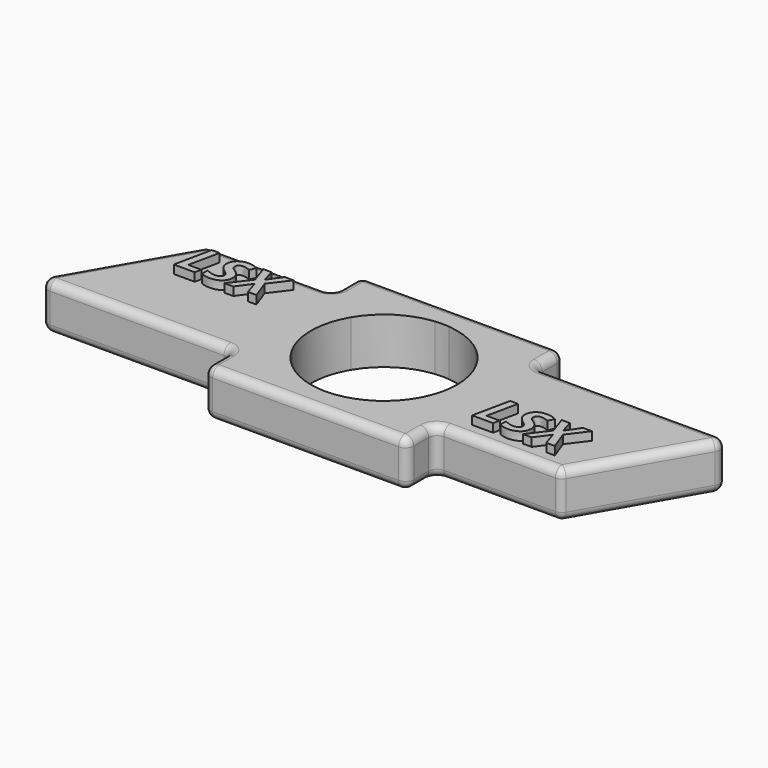
from build123d import *

# Parameters (mm, degrees)
F1_DEPTH     = 6.985
F2_TEXT_SIZE = 7.9375
F3_DEPTH     = 1.27
F4_R         = 1.27
F5_R         = 1.27
F6_R         = 1.27


# Not quite as in the source:
# - Text() gives the source's letters only with a copy of the font that has no kerning and outlines rounded to 1/6400 em; it was checked with that copy


with BuildPart() as f1:
    # F0 (on Top) → F1 (new body)
    with BuildSketch(Plane.XY):
        Polygon((-34.1459329325, 9.4483174), (-44.9994729931, -9.4487963283), (-15.3035, -9.4487963283), (-15.3035, -14.7827963283), (15.3035, -14.7827963283), (15.3035, -9.4487963283), (34.1459329325, -9.4487963283), (44.9994729931, 9.4483174), (15.3035, 9.4483174), (15.3035, 14.7823174), (-15.3035, 14.7823174), (-15.3035, 9.4483174), align=None)
        with BuildLine():
            Line((-11.4935, -5.6387963283), (-38.4175, -5.6387963283))
            Line((-38.4175, -5.6387963283), (-31.9405, 5.6383174))
            Line((-31.9405, 5.6383174), (-11.4935, 5.6383174))
            Line((-11.4935, 5.6383174), (-11.4935, 10.9723174))
            Line((-11.4935, 10.9723174), (-1.0620771317, 10.9723174))
            ThreePointArc((-1.0620771317, 10.9723174), (0, 11.0236), (1.0620771317, 10.9723174))
            Line((1.0620771317, 10.9723174), (11.4935, 10.9723174))
            Line((11.4935, 10.9723174), (11.4935, 5.6383174))
            Line((11.4935, 5.6383174), (38.4175, 5.6383174))
            Line((38.4175, 5.6383174), (31.9405, -5.6387963283))
            Line((31.9405, -5.6387963283), (11.4935, -5.6387963283))
            Line((11.4935, -5.6387963283), (11.4935, -10.9727963283))
            Line((11.4935, -10.9727963283), (1.0571176371, -10.9727963283))
            ThreePointArc((1.0571176371, -10.9727963283), (0, -11.0236), (-1.0571176371, -10.9727963283))
            Line((-1.0571176371, -10.9727963283), (-11.4935, -10.9727963283))
            Line((-11.4935, -10.9727963283), (-11.4935, -5.6387963283))
        make_face(mode=Mode.SUBTRACT)
        with BuildLine():
            Line((-31.9405, 5.6383174), (-38.4175, -5.6387963283))
            Line((-38.4175, -5.6387963283), (-11.4935, -5.6387963283))
            Line((-11.4935, -5.6387963283), (-11.4935, -10.9727963283))
            Line((-11.4935, -10.9727963283), (-1.0571176371, -10.9727963283))
            ThreePointArc((-1.0571176371, -10.9727963283), (-9.8336529635, -4.9818697649), (-9.4725463238, 5.6383174))
            Line((-9.4725463238, 5.6383174), (-11.4935, 5.6383174))
            Line((-11.4935, 5.6383174), (-31.9405, 5.6383174))
        make_face()
        with BuildLine():
            Line((-11.4935, 10.9723174), (-11.4935, 5.6383174))
            Line((-11.4935, 5.6383174), (-9.4725463238, 5.6383174))
            ThreePointArc((-9.4725463238, 5.6383174), (-5.9040208195, 9.30925857), (-1.0620771317, 10.9723174))
            Line((-1.0620771317, 10.9723174), (-11.4935, 10.9723174))
        make_face()
        with BuildLine():
            ThreePointArc((11.0236, 0), (8.1600551145, -7.4116973419), (1.0571176371, -10.9727963283))
            Line((1.0571176371, -10.9727963283), (11.4935, -10.9727963283))
            Line((11.4935, -10.9727963283), (11.4935, -5.6387963283))
            Line((11.4935, -5.6387963283), (31.9405, -5.6387963283))
            Line((31.9405, -5.6387963283), (38.4175, 5.6383174))
            Line((38.4175, 5.6383174), (11.4935, 5.6383174))
            Line((11.4935, 5.6383174), (11.4935, 10.9723174))
            Line((11.4935, 10.9723174), (1.0620771317, 10.9723174))
            ThreePointArc((1.0620771317, 10.9723174), (8.1617299156, 7.4098530178), (11.0236, 0))
        make_face()
    extrude(amount=F1_DEPTH)

    # F2 (on face) → F3 (join)
    with BuildSketch(Plane.XY.offset(6.985)):
        with Locations((-32.8759329325, 1.1933174)):
            Text('LSX', F2_TEXT_SIZE, font='Open Sans', font_style=FontStyle.BOLDITALIC, text_align=(TextAlign.LEFT, TextAlign.BOTTOM))
        with Locations((18.61323762, -6.9087963283)):
            Text('LSX', F2_TEXT_SIZE, font='Open Sans', font_style=FontStyle.BOLDITALIC, text_align=(TextAlign.LEFT, TextAlign.BOTTOM))
    extrude(amount=F3_DEPTH)

    # F4
    f4_edges = [f1.edges().sort_by_distance(p)[0] for p in [
        (-34.145933, 9.448317, 3.4925),
        (-15.3035, 14.782317, 3.4925),
        (15.3035, 14.782317, 3.4925),
        (15.3035, 9.448317, 3.4925),
        (44.999473, 9.448317, 3.4925),
        (15.3035, -14.782796, 3.4925),
        (15.3035, -9.448796, 3.4925),
        (34.145933, -9.448796, 3.4925),
        (-15.3035, -14.782796, 3.4925),
        (-44.999473, -9.448796, 3.4925),
        (-15.3035, -9.448796, 3.4925),
        (-15.3035, 9.448317, 3.4925),
    ]]
    fillet(f4_edges, radius=F4_R)

    # F5
    f5_edges = [f1.edges().sort_by_distance(p)[0] for p in [
        (-39.209416, 0.63228, 6.985),
    ]]
    fillet(f5_edges, radius=F5_R)

    # F6
    f6_edges = [f1.edges().sort_by_distance(p)[0] for p in [
        (-24.992144, 9.448317, 0),
    ]]
    fillet(f6_edges, radius=F6_R)


solid = f1.part
